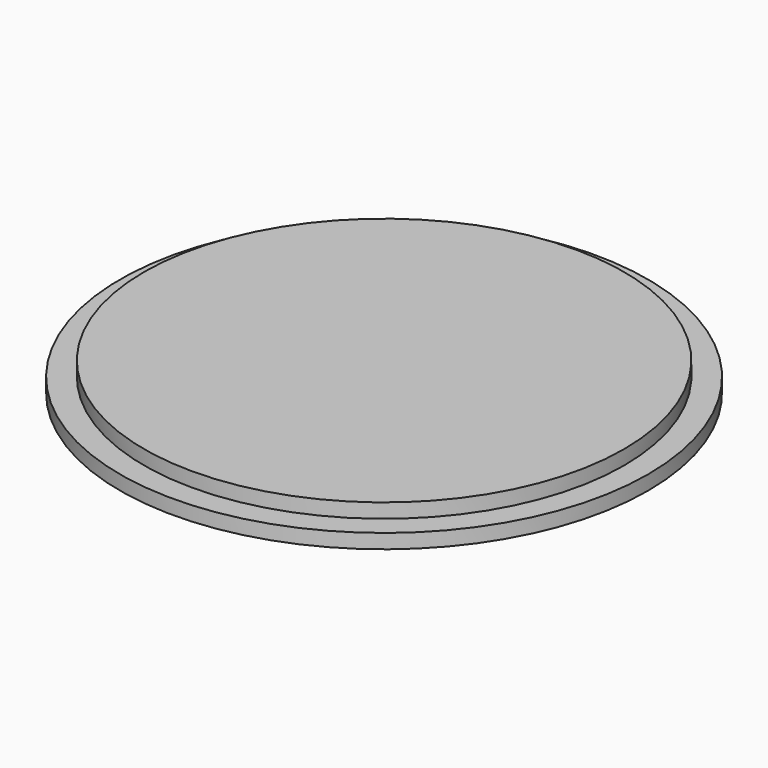
from build123d import *

# Parameters (mm, degrees)
F0_R     = 12.7
F1_DEPTH = 1.524
F2_R     = 13.97
F3_DEPTH = 0.762
F4_W     = 5.08
F4_H     = 1.524
F6_W     = 5.08000508
F6_H     = 1.5265774739
F7_DEPTH = 0.254
F8_R     = 0.25399


# Not quite as in the source:
# - a fillet or chamfer is up to 0.001 mm smaller than in the source, because OpenCascade refuses the exact size


with BuildPart() as f1:
    # F0 (on Top) → F1 (new body)
    with BuildSketch(Plane.XY):
        Circle(F0_R)
    extrude(amount=F1_DEPTH)

    # F2 (on Top) → F3 (join)
    with BuildSketch(Plane.XY):
        Circle(F2_R)
    extrude(amount=F3_DEPTH)

    # F4 (on Front) → F5 (revolve, cut)
    with BuildSketch(Plane.XZ):
        Rectangle(F4_W, F4_H)
    revolve(axis=Axis((0, 0, -0.762), (-1, 0, 0)), mode=Mode.SUBTRACT)

    # F6 (on Top) → F7 (join)
    with BuildSketch(Plane.XY):
        Rectangle(F6_W, F6_H)
    extrude(amount=F7_DEPTH)

    # F8 (radius 0.254 in the source; OpenCascade refuses exactly that, so slightly less here)
    f8_edges = [f1.edges().sort_by_distance(p)[0] for p in [
        (0, 0.763289, 0.254),
        (0, -0.763289, 0.254),
    ]]
    fillet(f8_edges, radius=F8_R)


solid = f1.part
